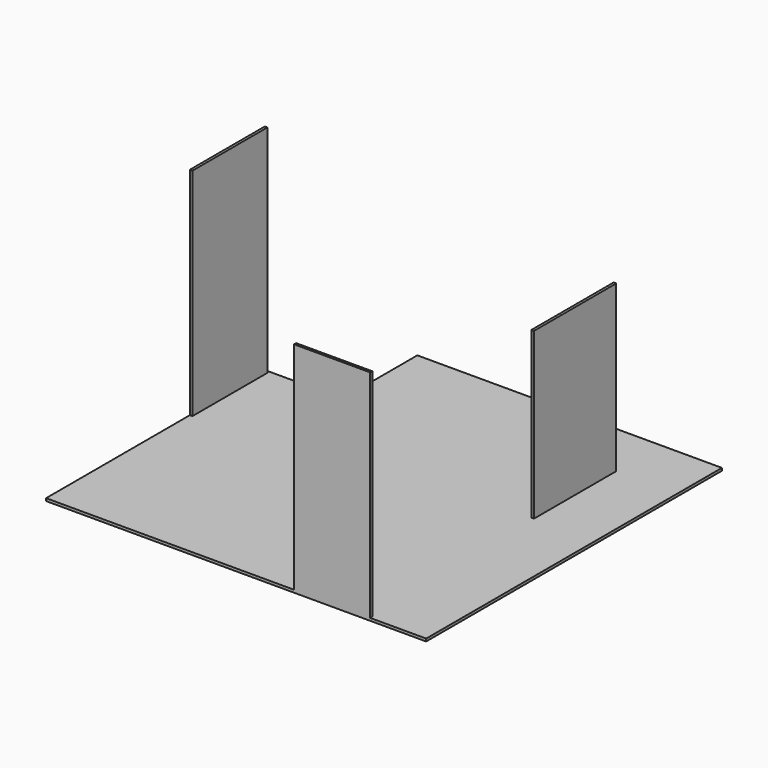
from build123d import *

# Parameters (mm, degrees)
F2_DEPTH = 25.4
F3_W     = 914.4
F3_H     = 2133.6
F4_DEPTH = 25.4
F5_W     = 742.95
F5_H     = 2133.6
F6_DEPTH = 25.4
F7_W     = 1003.3
F7_H     = 1612.9
F8_DEPTH = 25.4


with BuildPart() as f2:
    # F0 (on Top) → F2 (new body)
    with BuildSketch(Plane.XY):
        Polygon((0, 2692.4), (0, 0), (3708.4, 0), (3708.4, 3606.8), (736.6, 3606.8), (736.6, 2692.4), align=None)
    extrude(amount=F2_DEPTH)

    # F3 (on face) → F4 (join)
    with BuildSketch(Plane(origin=(0, 0, 0), x_dir=(0, -1, 0), z_dir=(-1, 0, 0))):
        with Locations((-2209.8, 1066.8)):
            Rectangle(F3_W, F3_H)
    extrude(amount=-F4_DEPTH)

    # F5 (on face) → F6 (join)
    with BuildSketch(Plane.XZ):
        with Locations((2790.825, 1066.8)):
            Rectangle(F5_W, F5_H)
    extrude(amount=-F6_DEPTH)


with BuildPart() as f8:
    # F7 (on face) → F8 (new body)
    with BuildSketch(Plane.YZ.offset(3708.4)):
        with Locations((1816.1, 1327.15)):
            Rectangle(F7_W, F7_H)
    extrude(amount=-F8_DEPTH)


solid = Compound([f2.part, f8.part])
